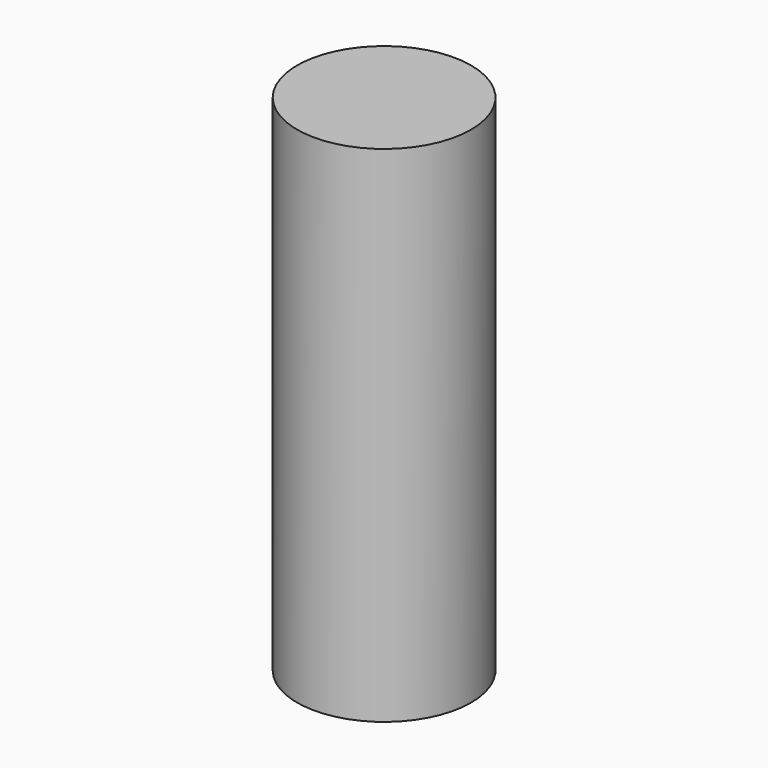
from build123d import *

# Parameters (mm, degrees)
F0_R     = 28.6512
F1_DEPTH = 83.058
F2_W     = 18.0594
F2_H     = 15.9512
F4_DEPTH = 60.706


# Not quite as in the source:
# - a feature of the source that left no trace in its solid (it failed there, or was rolled back) is left out


with BuildPart() as f1:
    # F0 (on Top) → F1 (new body, symmetric)
    with BuildSketch(Plane.XY):
        Circle(F0_R)
    extrude(amount=F1_DEPTH, both=True)

    # F2 (on Right) → F4 (cut)
    with BuildSketch(Plane.YZ):
        with Locations((9.0297, 7.9756)):
            Rectangle(F2_W, F2_H)
    extrude(amount=-F4_DEPTH, mode=Mode.SUBTRACT)


solid = f1.part
